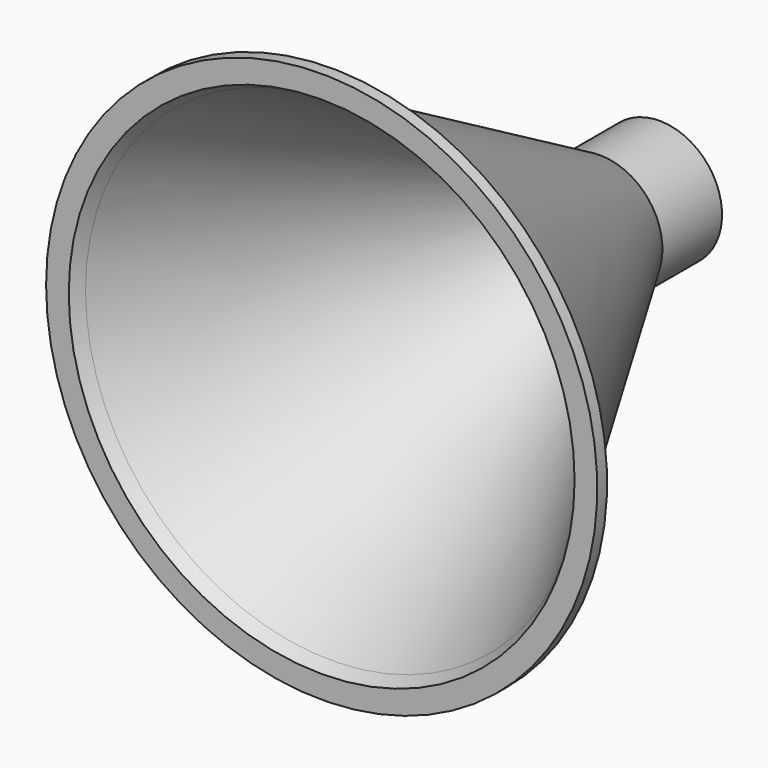
from build123d import *

# Parameters (mm, degrees)
F4_DEPTH = 3


with BuildPart() as f1:
    # F0 (on Top) → F1 (revolve)
    with BuildSketch(Plane.XY):
        Polygon((-41.3627406567, 2), (-40.1627406567, 2), (-7.2, 59.9687313223), (-8.4, 59.9687313223), (-10.2, 56.8032264431), align=None)
        Polygon((-10.2, 56.8032264431), (-8.4, 59.9687313223), (-10.2, 59.9687313223), align=None)
        Polygon((-8.4, 59.9687313223), (-7.2, 59.9687313223), (-7.2, 68.9687313223), (-10.2, 68.9687313223), (-10.2, 59.9687313223), align=None)
        Polygon((-42.5, 0), (-41.3, 0), (-40.1627406567, 2), (-41.3627406567, 2), align=None)
        Polygon((-45, 0), (-42.5, 0), (-41.3627406567, 2), (-45, 2), align=None)
    revolve(axis=Axis((0, 36.8, 0), (0, 1, 0)))

    # F3 (on offset) → F4 (join)
    with BuildSketch(Plane(origin=(0, 68.9687313223, 0), x_dir=(-1, 0, 0), z_dir=(0, 1, 0))):
        with BuildLine():
            ThreePointArc((6.2, -3.6606010435), (6.9455021417, -1.8973665961), (7.2, 0))
            ThreePointArc((7.2, 0), (6.9455021417, 1.8973665961), (6.2, 3.6606010435))
            Line((6.2, 3.6606010435), (6.2, 0))
            Line((6.2, 0), (6.2, -3.6606010435))
        make_face()
        with BuildLine():
            Line((-6.2, -3.6606010435), (-6.2, 3.6606010435))
            ThreePointArc((-6.2, 3.6606010435), (-7.2, 0), (-6.2, -3.6606010435))
        make_face()
    extrude(amount=-F4_DEPTH)


solid = f1.part
